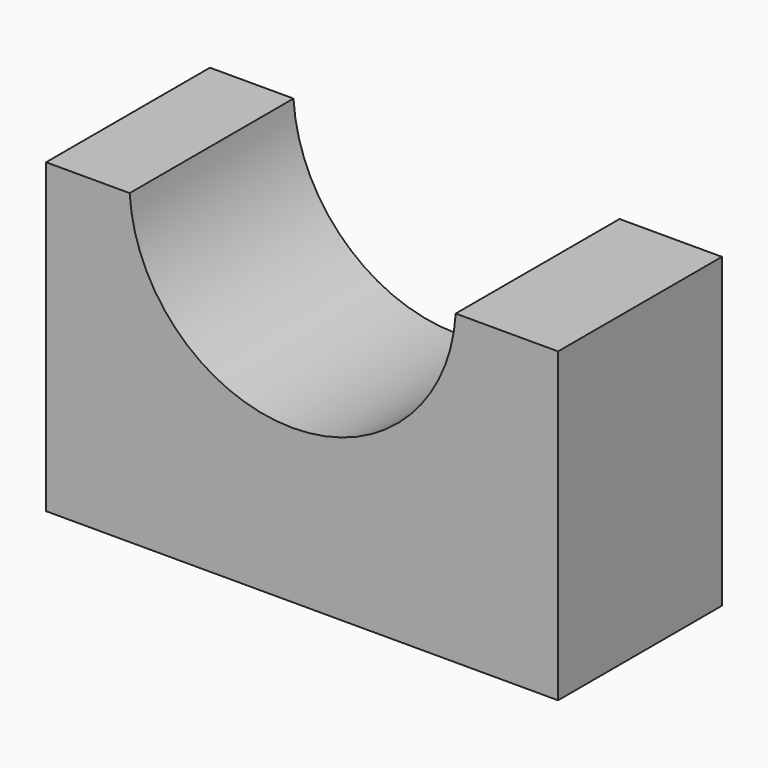
from build123d import *

# Parameters (mm, degrees)
F0_W     = 63.5
F0_H     = 38.1
F1_DEPTH = 25.4
F3_DEPTH = 25.401


with BuildPart() as f1:
    # F0 (on Front) → F1 (new body)
    with BuildSketch(Plane.XZ):
        with Locations((-31.75, 19.05)):
            Rectangle(F0_W, F0_H)
    extrude(amount=F1_DEPTH)

    # F2 (on face) → F3 (cut, through all)
    with BuildSketch(Plane.XZ.offset(25.4)):
        with BuildLine():
            Line((-12.7, 38.1), (-53.134321885, 38.1))
            ThreePointArc((-53.134321885, 38.1), (-32.9171609425, 19.0326653727), (-12.7, 38.1))
        make_face()
    extrude(amount=-F3_DEPTH, mode=Mode.SUBTRACT)


solid = f1.part
